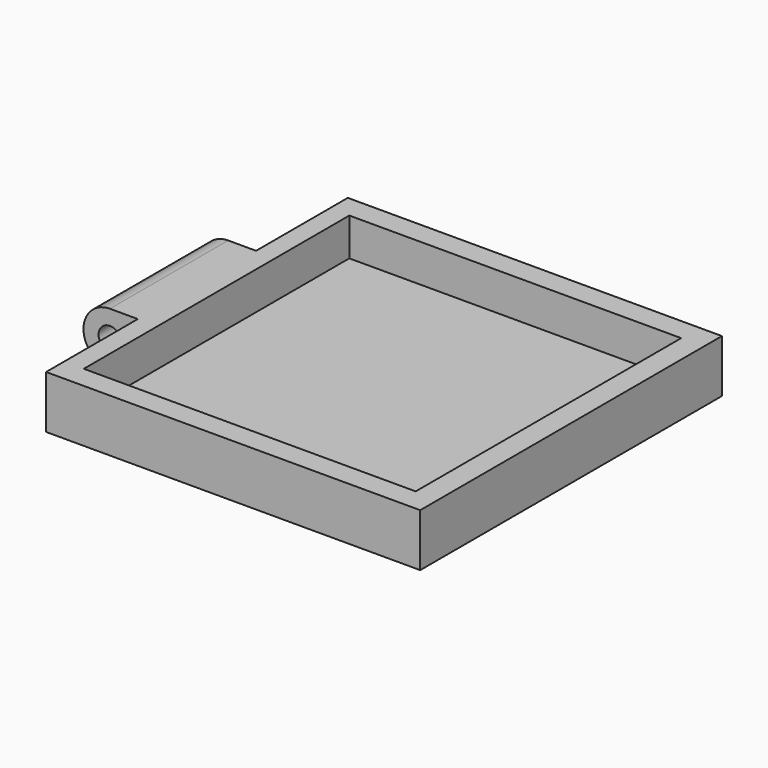
from build123d import *

# Parameters (mm, degrees)
F1_DEPTH = 7
F2_R     = 3.49999
F4_D     = 3
F5_W     = 44
F5_H     = 44
F6_DEPTH = 5


# Not quite as in the source:
# - a fillet or chamfer is up to 0.001 mm smaller than in the source, because OpenCascade refuses the exact size


with BuildPart() as f1:
    # F0 (on Top) → F1 (new body)
    with BuildSketch(Plane.XY):
        Polygon((28.4, 25), (-21.2, 25), (-21.2, 9.8), (-28.4, 9.8), (-28.4, -9.8), (-21.2, -9.8), (-21.2, -25), (28.4, -25), align=None)
    extrude(amount=F1_DEPTH)

    # F2 (radius 3.5 in the source; OpenCascade refuses exactly that, so slightly less here)
    f2_edges = [f1.edges().sort_by_distance(p)[0] for p in [
        (-28.4, 0, 7),
        (-28.4, 0, 0),
    ]]
    fillet(f2_edges, radius=F2_R)

    # F4 (through all)
    with Locations(Plane(origin=(0, 9.8, 0), x_dir=(-1, 0, 0), z_dir=(0, 1, 0))):
        with Locations((24.9, 3.5)):
            Hole(F4_D / 2)

    # F5 (on face) → F6 (cut)
    with BuildSketch(Plane.XY.offset(7)):
        with Locations((3.4, 0)):
            Rectangle(F5_W, F5_H)
    extrude(amount=-F6_DEPTH, mode=Mode.SUBTRACT)


solid = f1.part
